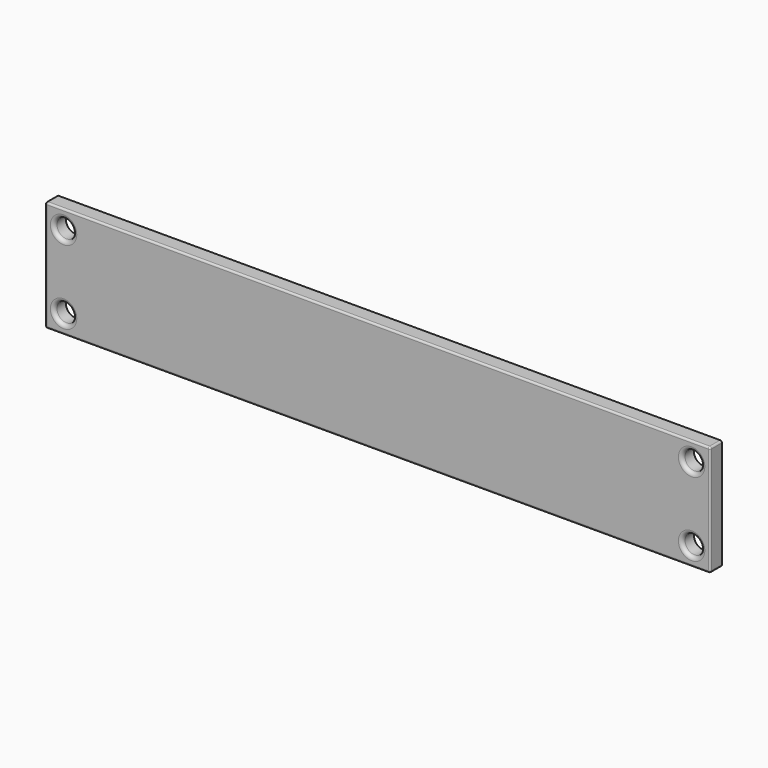
from build123d import *

# Parameters (mm, degrees)
F0_W         = 180
F0_H         = 30
F0_R         = 2.5751263091
F1_DEPTH     = 4
F2_R         = 1
F3_R         = 0.5
F4_TEXT_SIZE = 7.4360960496
F5_DEPTH     = 1


# Not quite as in the source:
# - a feature names something its author has since deleted; it is built from what else it names
# - Text() gives the source's letters only with a copy of the font that has no kerning and outlines rounded to 1/6400 em; it was checked with that copy


with BuildPart() as f1:
    # F0 (on Front) → F1 (new body)
    with BuildSketch(Plane.XZ):
        Rectangle(F0_W, F0_H)
        with Locations((-85, -10)):
            Circle(F0_R, mode=Mode.SUBTRACT)
        with Locations((85, -10)):
            Circle(F0_R, mode=Mode.SUBTRACT)
        with Locations((-85, 10)):
            Circle(F0_R, mode=Mode.SUBTRACT)
        with Locations((85, 10)):
            Circle(F0_R, mode=Mode.SUBTRACT)
    extrude(amount=F1_DEPTH)

    # F2
    f2_edges = [f1.edges().sort_by_distance(p)[0] for p in [
        (-87.575126, -4, 10),
        (-87.575126, -4, -10),
        (82.424874, -4, 10),
        (82.424874, -4, -10),
    ]]
    fillet(f2_edges, radius=F2_R)

    # F3
    f3_edges = [f1.edges().sort_by_distance(p)[0] for p in [
        (0, -4, 15),
        (-90, -4, 0),
        (0, -4, -15),
        (90, -4, 0),
        (-90, -2, 15),
        (-90, -2, -15),
        (90, -2, 15),
        (90, -2, -15),
    ]]
    fillet(f3_edges, radius=F3_R)

    # F4 (on face) → F5 (join)
    with BuildSketch(Plane(origin=(0, 0, 0), x_dir=(-1, 0, 0), z_dir=(0, 1, 0))):
        with Locations((-70.7097770646, -2.4972305579)):
            Text('Tetra Stylus Body', F4_TEXT_SIZE, font='Open Sans', text_align=(TextAlign.LEFT, TextAlign.BOTTOM))
    extrude(amount=F5_DEPTH)

    # F6: F1 across plane


with BuildPart() as f1_1:
    add(f1.part)
    add(f1.part.mirror(Plane.YZ))


solid = f1_1.part
